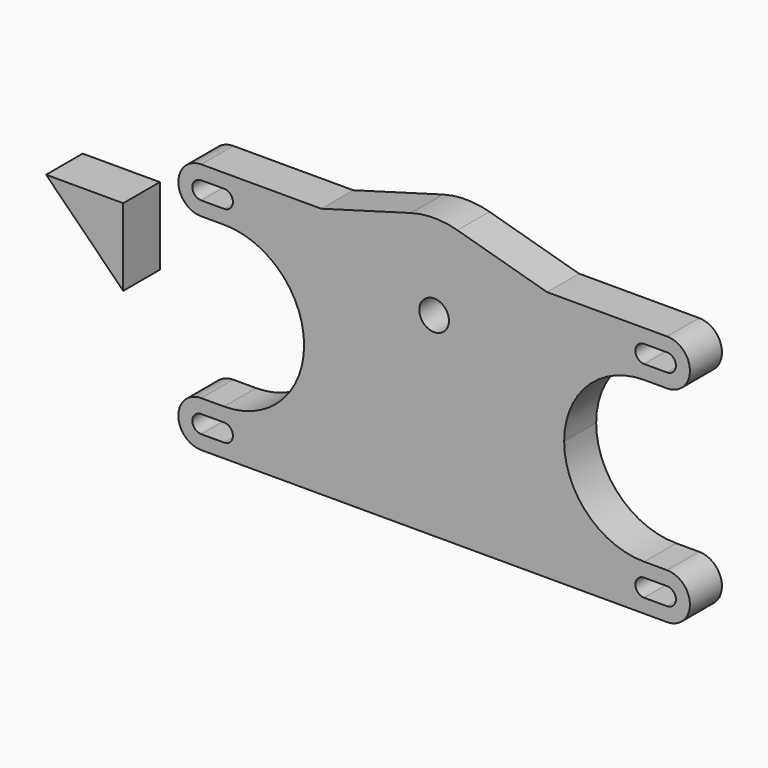
from build123d import *

# Parameters (mm, degrees)
F0_R          = 2.6
F1_DEPTH      = 3.5
F1_DEPTH_BACK = 3.5
F2_DEPTH      = 8
F3_R          = 3


# Not quite as in the source:
# - ends of sketch curves that miss each other by under 0.0002 mm in the source are joined


with BuildPart() as f1:
    # F0 (on Front) → F1 (new body, two sides)
    with BuildSketch(Plane.XZ) as f1_sk:
        with BuildLine():
            Line((40.7500048285, 7.4198008843), (19.75, 7.4198008843))
            Line((19.75, 7.4198008843), (19.75, -14.5801991157))
            Line((19.75, -14.5801991157), (22.7499971869, -14.5801991157))
            ThreePointArc((22.7499971869, -14.5801991157), (26.8505050634, -4.6807041791), (36.75, -0.5801991157))
            Line((36.75, -0.5801991157), (40.75, -0.5801991157))
            ThreePointArc((40.75, -0.5801991157), (44.75, 3.4197984701), (40.7500048285, 7.4198008843))
        make_face()
        with BuildLine():
            Line((40.75, 1.8698008843), (36.75, 1.8698008843))
            ThreePointArc((36.75, 1.8698008843), (35.2, 3.4198008843), (36.75, 4.9698008843))
            Line((36.75, 4.9698008843), (40.75, 4.9698008843))
            ThreePointArc((40.75, 4.9698008843), (42.3, 3.4198008843), (40.75, 1.8698008843))
        make_face(mode=Mode.SUBTRACT)
        with BuildLine():
            Line((22.7499971869, -14.5801991157), (19.75, -14.5801991157))
            Line((19.75, -14.5801991157), (19.75, -36.5801991157))
            Line((19.75, -36.5801991157), (40.7500048285, -36.5801991157))
            ThreePointArc((40.7500048285, -36.5801991157), (44.75, -32.5801967015), (40.75, -28.5801991157))
            Line((40.75, -28.5801991157), (36.75, -28.5801991157))
            ThreePointArc((36.75, -28.5801991157), (26.8505050634, -24.4796940523), (22.7499971869, -14.5801991157))
        make_face()
        with BuildLine():
            ThreePointArc((40.75, -31.0301991157), (42.3, -32.5801991157), (40.75, -34.1301991157))
            Line((40.75, -34.1301991157), (36.75, -34.1301991157))
            ThreePointArc((36.75, -34.1301991157), (35.2, -32.5801991157), (36.75, -31.0301991157))
            Line((36.75, -31.0301991157), (40.75, -31.0301991157))
        make_face(mode=Mode.SUBTRACT)
        with BuildLine():
            ThreePointArc((4.0844565269, 11.8529992436), (11.9638381781, 6.4678159179), (15, -2.5801991157))
            ThreePointArc((15, -2.5801991157), (-9.0480150336, -14.5440372938), (-4.0844565269, 11.8529992436))
            Line((-4.0844565269, 11.8529992436), (-19.75, 7.4198008843))
            Line((-19.75, 7.4198008843), (-19.75, -14.5801991157))
            Line((-19.75, -14.5801991157), (-19.75, -36.5801991157))
            Line((-19.75, -36.5801991157), (0, -36.5801991157))
            Line((0, -36.5801991157), (19.75, -36.5801991157))
            Line((19.75, -36.5801991157), (19.75, -14.5801991157))
            Line((19.75, -14.5801991157), (19.75, 7.4198008843))
            Line((19.75, 7.4198008843), (4.0844565269, 11.8529992436))
        make_face()
        with BuildLine():
            ThreePointArc((-4.0844565269, 11.8529992436), (-9.0480150336, -14.5440372938), (15, -2.5801991157))
            ThreePointArc((15, -2.5801991157), (11.9638381781, 6.4678159179), (4.0844565269, 11.8529992436))
            ThreePointArc((4.0844565269, 11.8529992436), (0, 12.4198008843), (-4.0844565269, 11.8529992436))
        make_face()
        with Locations((0, -2.5801991157)):
            Circle(F0_R, mode=Mode.SUBTRACT)
        with BuildLine():
            Line((-19.75, -14.5801991157), (-19.75, 7.4198008843))
            Line((-19.75, 7.4198008843), (-40.7500048285, 7.4198008843))
            ThreePointArc((-40.7500048285, 7.4198008843), (-44.75, 3.4197984701), (-40.75, -0.5801991157))
            Line((-40.75, -0.5801991157), (-36.75, -0.5801991157))
            ThreePointArc((-36.75, -0.5801991157), (-26.8505050634, -4.6807041791), (-22.75, -14.5801991157))
            Line((-22.75, -14.5801991157), (-19.75, -14.5801991157))
        make_face()
        with BuildLine():
            ThreePointArc((-36.75, 4.9698008843), (-35.2, 3.4198008843), (-36.75, 1.8698008843))
            Line((-36.75, 1.8698008843), (-40.75, 1.8698008843))
            ThreePointArc((-40.75, 1.8698008843), (-42.3, 3.4198008843), (-40.75, 4.9698008843))
            Line((-40.75, 4.9698008843), (-36.75, 4.9698008843))
        make_face(mode=Mode.SUBTRACT)
        with BuildLine():
            Line((-19.75, -36.5801991157), (-19.75, -14.5801991157))
            Line((-19.75, -14.5801991157), (-22.7499971869, -14.5801991157))
            ThreePointArc((-22.7499971869, -14.5801991157), (-26.8505050634, -24.4796940523), (-36.75, -28.5801991157))
            Line((-36.75, -28.5801991157), (-40.75, -28.5801991157))
            ThreePointArc((-40.75, -28.5801991157), (-44.75, -32.5801967015), (-40.7500048285, -36.5801991157))
            Line((-40.7500048285, -36.5801991157), (-19.75, -36.5801991157))
        make_face()
        with BuildLine():
            Line((-36.75, -34.1301991157), (-40.75, -34.1301991157))
            ThreePointArc((-40.75, -34.1301991157), (-42.3, -32.5801991157), (-40.75, -31.0301991157))
            Line((-40.75, -31.0301991157), (-36.75, -31.0301991157))
            ThreePointArc((-36.75, -31.0301991157), (-35.2, -32.5801991157), (-36.75, -34.1301991157))
        make_face(mode=Mode.SUBTRACT)
    extrude(amount=F1_DEPTH)
    extrude(f1_sk.sketch, amount=-F1_DEPTH_BACK)

    # F3 (on Right) → F4 (revolve, cut)
    with BuildSketch(Plane.YZ):
        with Locations((4, 7.4198008843)):
            Circle(F3_R)
    revolve(axis=Axis((0, 0, -2.5801991157), (0, -1, 0)), mode=Mode.SUBTRACT)


with BuildPart() as f2:
    # F0 (on Front) → F2 (new body)
    with BuildSketch(Plane.XZ):
        Polygon((-50.7889514565, -13.5), (-50.7889514565, 0), (-64.2889514565, 0), align=None)
    extrude(amount=F2_DEPTH)


solid = Compound([f1.part, f2.part])
